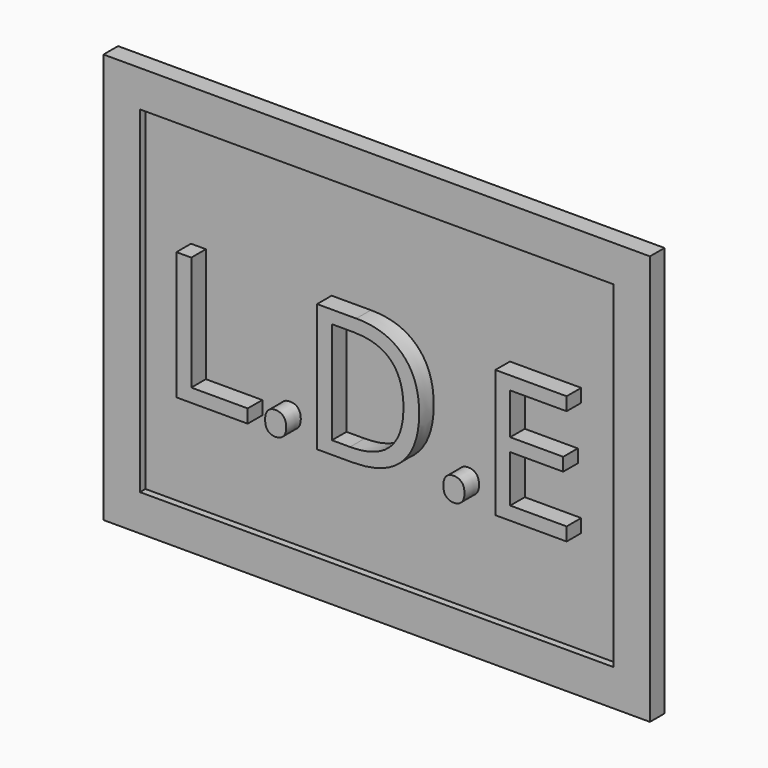
from build123d import *

# Parameters (mm, degrees)
F0_W          = 600
F0_H          = 20
F1_DEPTH      = 450
F2_W          = 520
F2_H          = 370
F3_DEPTH      = 25
F5_W          = 320
F5_H          = 230
F6_DEPTH      = 42.5615510906
F7_SIZE       = 15
F8_R          = 14
F9_DEPTH      = 25
F11_TEXT_SIZE = 196.6807163424
F12_DEPTH     = 20


# Not quite as in the source:
# - Text() gives the source's letters only with a copy of the font that has no kerning and outlines rounded to 1/6400 em; it was checked with that copy


with BuildPart() as f1:
    # F0 (on Top) → F1 (new body)
    with BuildSketch(Plane.XY):
        with Locations((0, 27.4384489094)):
            Rectangle(F0_W, F0_H)
    extrude(amount=F1_DEPTH)

    # F2 (on Front) → F3 (cut)
    with BuildSketch(Plane.XZ):
        with Locations((0, 225)):
            Rectangle(F2_W, F2_H)
    extrude(amount=-F3_DEPTH, mode=Mode.SUBTRACT)

    # F5 (on offset) → F6 (join, through all)
    with BuildSketch(Plane.XZ.offset(-80)):
        with Locations((0, 225)):
            Rectangle(F5_W, F5_H)
    extrude(amount=F6_DEPTH)

    # F7
    f7_edges = [f1.edges().sort_by_distance(p)[0] for p in [
        (160, 80, 225),
        (0, 80, 340),
        (-160, 80, 225),
        (0, 80, 110),
    ]]
    chamfer(f7_edges, length=F7_SIZE)

    # F8 (on offset) → F9 (cut)
    with BuildSketch(Plane.XZ.offset(-80)):
        with Locations((0, 225)):
            Circle(F8_R)
    extrude(amount=F9_DEPTH, mode=Mode.SUBTRACT)

    # F11 (on offset) → F12 (join, through all)
    with BuildSketch(Plane.XZ.offset(-5)):
        with Locations((-229.2529568076, 152.9166251421)):
            Text('L.D.E', F11_TEXT_SIZE, font='Open Sans', text_align=(TextAlign.LEFT, TextAlign.BOTTOM))
    extrude(amount=-F12_DEPTH)


solid = f1.part
